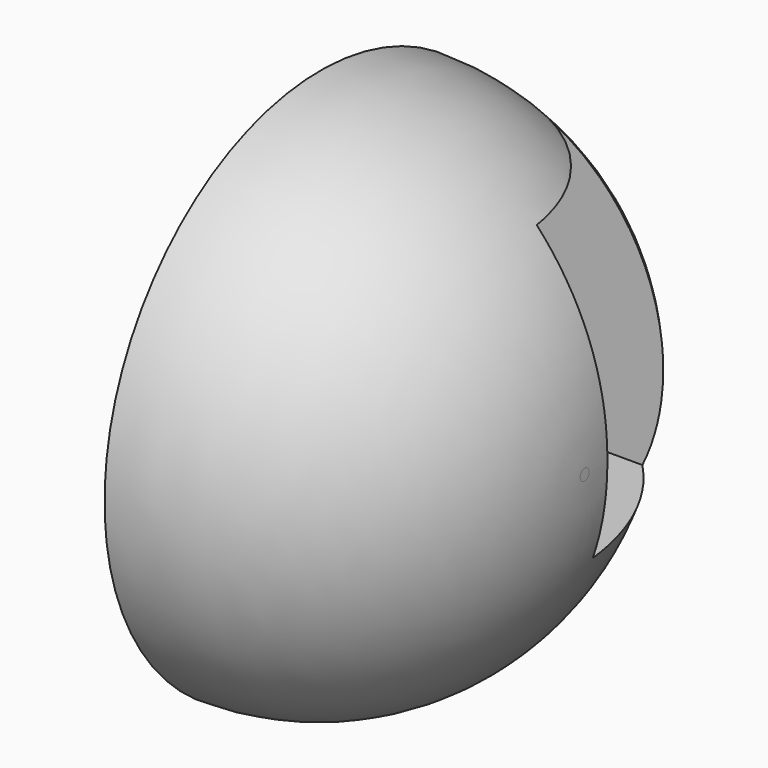
from build123d import *

# Parameters (mm, degrees)
F1_R      = 23.5
F2_DEPTH  = 23
F3_R      = 22.99999
F0_W      = 32
F0_H      = 31.9999990161
F4_DEPTH  = 3
F5_R      = 2.25
F6_DEPTH  = 8
F7_W      = 12.7981919795
F7_H      = 23.941071704
F8_DEPTH  = 23.001
F9_W      = 11.722983385
F9_H      = 16.8361999094
F10_DEPTH = 13


# Not quite as in the source:
# - a fillet or chamfer is up to 0.001 mm smaller than in the source, because OpenCascade refuses the exact size


with BuildPart() as f2:
    # F1 (on Right) → F2 (new body)
    with BuildSketch(Plane.YZ):
        Circle(F1_R)
    extrude(amount=F2_DEPTH)

    # F3 (radius 23 in the source; OpenCascade refuses exactly that, so slightly less here)
    f3_edges = [f2.edges().sort_by_distance(p)[0] for p in [
        (23, -23.5, 0),
    ]]
    fillet(f3_edges, radius=F3_R)

    # F0 (on Right) → F4 (cut)
    with BuildSketch(Plane.YZ):
        with Locations((-0.437150538, 0.2656796428)):
            Rectangle(F0_W, F0_H)
    extrude(amount=F4_DEPTH, mode=Mode.SUBTRACT)

    # F5 (on Right) → F6 (cut)
    with BuildSketch(Plane.YZ):
        with Locations((18.515, 0)):
            Circle(F5_R)
        with Locations((-19.4516796619, 0)):
            Circle(F5_R)
    extrude(amount=F6_DEPTH, mode=Mode.SUBTRACT)

    # F7 (on face) → F8 (cut, through all)
    with BuildSketch(Plane.YZ):
        with Locations((8.9887827635, 4.0837647393)):
            Rectangle(F7_W, F7_H)
    extrude(amount=F8_DEPTH, mode=Mode.SUBTRACT)

    # F9 (on Right) → F10 (cut)
    with BuildSketch(Plane.YZ):
        with Locations((-6.7771898757, 4.8962011933)):
            Rectangle(F9_W, F9_H)
    extrude(amount=F10_DEPTH, mode=Mode.SUBTRACT)


solid = f2.part
